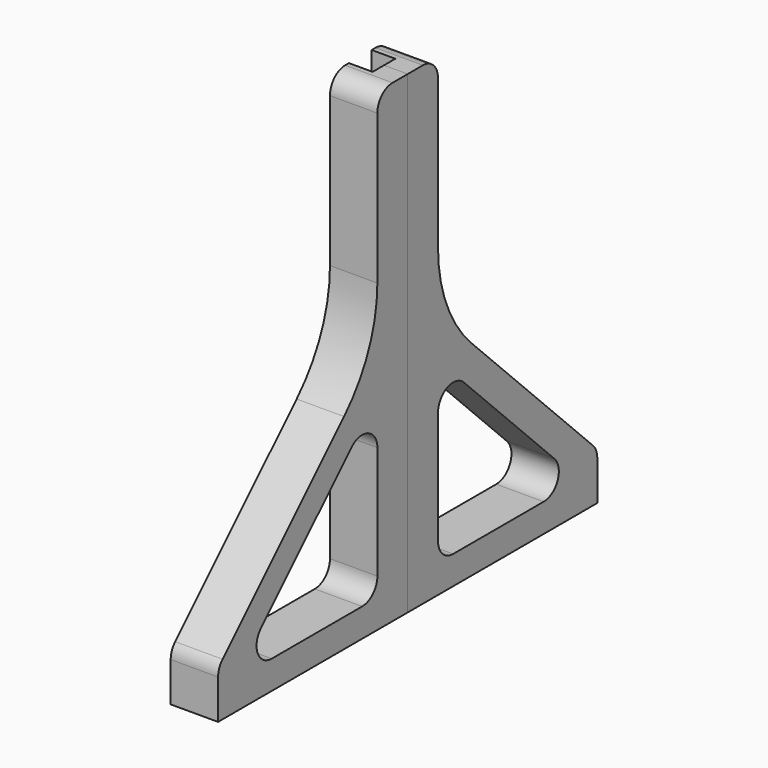
from build123d import *

# Parameters (mm, degrees)
F2_DEPTH = 2.5
F3_R     = 2
F3_2_R   = 2
F4_R     = 15
F4_2_R   = 15
F6_W     = 2.5
F6_H     = 3
F7_DEPTH = 47.001


# Not quite as in the source:
# - a pattern or mirror of a feature is missing from the dataset's text; its kind, count and spacing are read off the source's solid


with BuildPart() as f2:
    # F1 (on offset) → F2 (new body, symmetric)
    with BuildSketch(Plane.YZ.offset(55.5)):
        Polygon((0, 0), (25, 0), (25, 5), (4, 26), (4, 50), (0, 50), align=None)
        Polygon((4, 3), (4, 21.7573593129), (22.7573593129, 3), align=None, mode=Mode.SUBTRACT)
    extrude(amount=F2_DEPTH, both=True)


with BuildPart() as f2_copies_1:
    # F2_copies: instance of F2
    add(f2.part.mirror(Plane(origin=(0, 0, 0), x_dir=(0, 0, -1), z_dir=(0, -1, 0))))

    # F3#2
    f3_2_edges = [f2_copies_1.edges().sort_by_distance(p)[0] for p in [
        (55.5, -4, 50),
        (55.5, -25, 5),
        (55.5, -4, 21.757359),
        (55.5, -22.757359, 3),
        (55.5, -4, 3),
    ]]
    fillet(f3_2_edges, radius=F3_2_R)

    # F4#2
    f4_2_edges = [f2_copies_1.edges().sort_by_distance(p)[0] for p in [
        (55.5, -4, 26),
    ]]
    fillet(f4_2_edges, radius=F4_2_R)


with BuildPart() as f2_1:
    add(f2.part)

    # F3
    f3_edges = [f2_1.edges().sort_by_distance(p)[0] for p in [
        (55.5, 4, 50),
        (55.5, 25, 5),
        (55.5, 22.757359, 3),
        (55.5, 4, 3),
        (55.5, 4, 21.757359),
    ]]
    fillet(f3_edges, radius=F3_R)

    # F4
    f4_edges = [f2_1.edges().sort_by_distance(p)[0] for p in [
        (55.5, 4, 26),
    ]]
    fillet(f4_edges, radius=F4_R)


with BuildPart() as f7_tool:
    # F6 (on offset) → F7 (new body, through all)
    with BuildSketch(Plane.XY.offset(3)):
        with Locations((54.25, 0)):
            Rectangle(F6_W, F6_H)
    extrude(amount=F7_DEPTH)


with BuildPart() as f2_2:
    add(f2_1.part)

    # F7: cut by f7_tool
    add(f7_tool.part, mode=Mode.SUBTRACT)


with BuildPart() as f2_copies_1_1:
    add(f2_copies_1.part)

    # F7: cut by f7_tool
    add(f7_tool.part, mode=Mode.SUBTRACT)


solid = Compound([f2_2.part, f2_copies_1_1.part])
